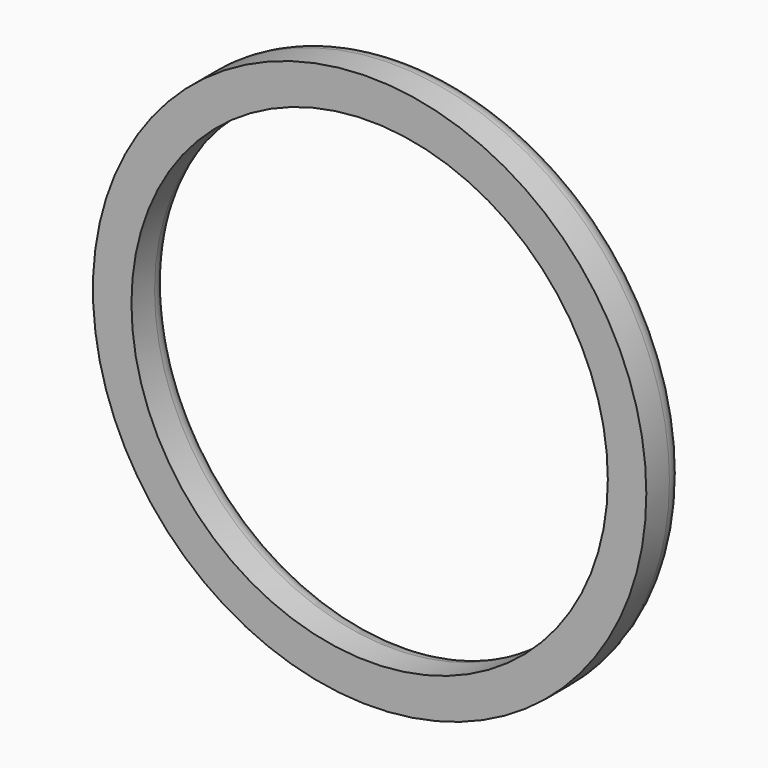
from build123d import *

# Parameters (mm, degrees)
F0_R     = 11.5
F0_R_2   = 9.9
F1_DEPTH = 2
F2_R     = 0.79999


# Not quite as in the source:
# - a fillet or chamfer is up to 0.001 mm smaller than in the source, because OpenCascade refuses the exact size


with BuildPart() as f1:
    # F0 (on Front) → F1 (new body)
    with BuildSketch(Plane.XZ):
        Circle(F0_R)
        Circle(F0_R_2, mode=Mode.SUBTRACT)
    extrude(amount=F1_DEPTH)

    # F2 (radius 0.8 in the source; OpenCascade refuses exactly that, so slightly less here)
    f2_edges = [f1.edges().sort_by_distance(p)[0] for p in [
        (-11.5, 0, 0),
        (-9.9, 0, 0),
    ]]
    fillet(f2_edges, radius=F2_R)


solid = f1.part
